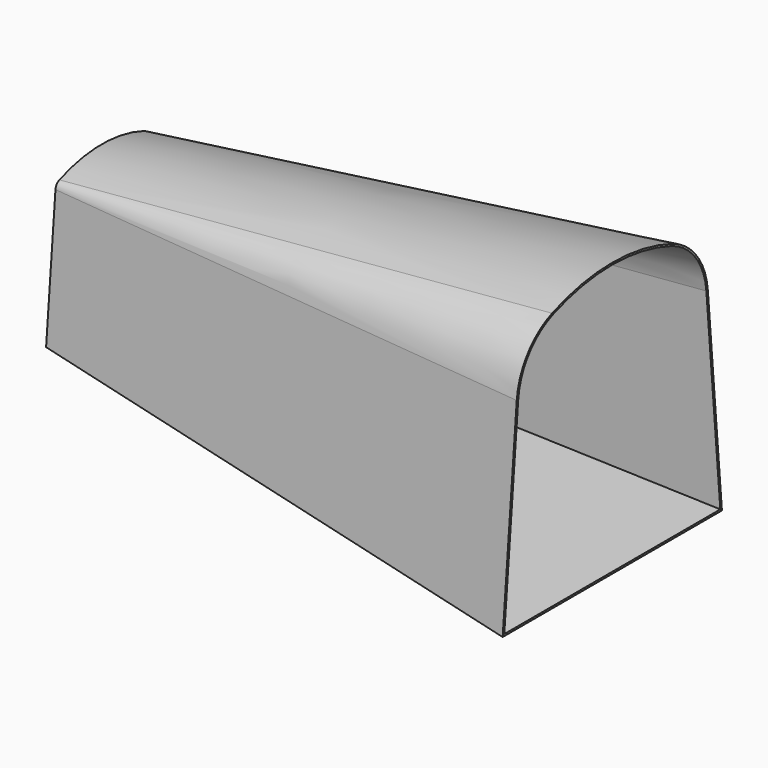
from build123d import *

# Parameters (mm, degrees)
F1_DEPTH               = 1676.4
F1_TAPER               = -6.9
F2_DEPTH               = 1676.4
DRAFT_F2_DRAFTED_ANGLE = -6.91


# Not quite as in the source:
# - an extrude with a draft is written as a straight extrude whose walls are then drafted


with BuildPart() as f1:
    # F0 (on Right) → F1 (new body)
    with BuildSketch(Plane.YZ):
        with BuildLine():
            Line((-190.1066201265, 439.9813452645), (-228.6, 0))
            Line((-228.6, 0), (228.6, 0))
            Line((228.6, 0), (190.1066201265, 439.9813452645))
            ThreePointArc((190.1066201265, 439.9813452645), (185.1057558503, 453.030920064), (173.9590122835, 461.460045393))
            ThreePointArc((173.9590122835, 461.460045393), (0, 493.9033815022), (-173.9590122835, 461.460045393))
            ThreePointArc((-173.9590122835, 461.460045393), (-185.1057558503, 453.030920064), (-190.1066201265, 439.9813452645))
        make_face()
        with BuildLine():
            Line((183.7323641581, 439.9813452645), (221.6701910182, 6.35))
            Line((221.6701910182, 6.35), (-221.6701910182, 6.35))
            Line((-221.6701910182, 6.35), (-183.7323641581, 439.9813452645))
            ThreePointArc((-183.7323641581, 439.9813452645), (-179.9896947319, 449.5336921504), (-171.6700779114, 455.5369313944))
            ThreePointArc((-171.6700779114, 455.5369313944), (0, 487.5533815022), (171.6700779114, 455.5369313944))
            ThreePointArc((171.6700779114, 455.5369313944), (179.9896947319, 449.5336921504), (183.7323641581, 439.9813452645))
        make_face(mode=Mode.SUBTRACT)
    extrude(amount=F1_DEPTH, taper=F1_TAPER)


with BuildPart() as f2_drafted:
    # F0 (on Right) → F2 (new body)
    with BuildSketch(Plane.YZ):
        with BuildLine():
            Line((-221.6701910182, 6.35), (221.6701910182, 6.35))
            Line((221.6701910182, 6.35), (183.7323641581, 439.9813452645))
            ThreePointArc((183.7323641581, 439.9813452645), (179.9896947319, 449.5336921504), (171.6700779114, 455.5369313944))
            ThreePointArc((171.6700779114, 455.5369313944), (0, 487.5533815022), (-171.6700779114, 455.5369313944))
            ThreePointArc((-171.6700779114, 455.5369313944), (-179.9896947319, 449.5336921504), (-183.7323641581, 439.9813452645))
            Line((-183.7323641581, 439.9813452645), (-221.6701910182, 6.35))
        make_face()
    extrude(amount=F2_DEPTH)

    # draft_F2_drafted
    draft_f2_drafted_walls = [f2_drafted.faces().sort_by_distance(p)[0] for p in [
        (1117.6, -202.7012775881, 223.1656726323),
        (1117.6, 0, 6.35),
        (1117.6, 202.7012775881, 223.1656726323),
        (1117.6, 179.9896947319, 449.5336921504),
        (1117.6, 0, 487.5533815022),
        (1117.6, -179.9896947319, 449.5336921504),
    ]]
    draft(draft_f2_drafted_walls, neutral_plane=Plane.YZ, angle=DRAFT_F2_DRAFTED_ANGLE)


with BuildPart() as f1_1:
    add(f1.part)

    # join_F2_drafted: cut F2_drafted
    add(f2_drafted.part, mode=Mode.SUBTRACT)


solid = f1_1.part
